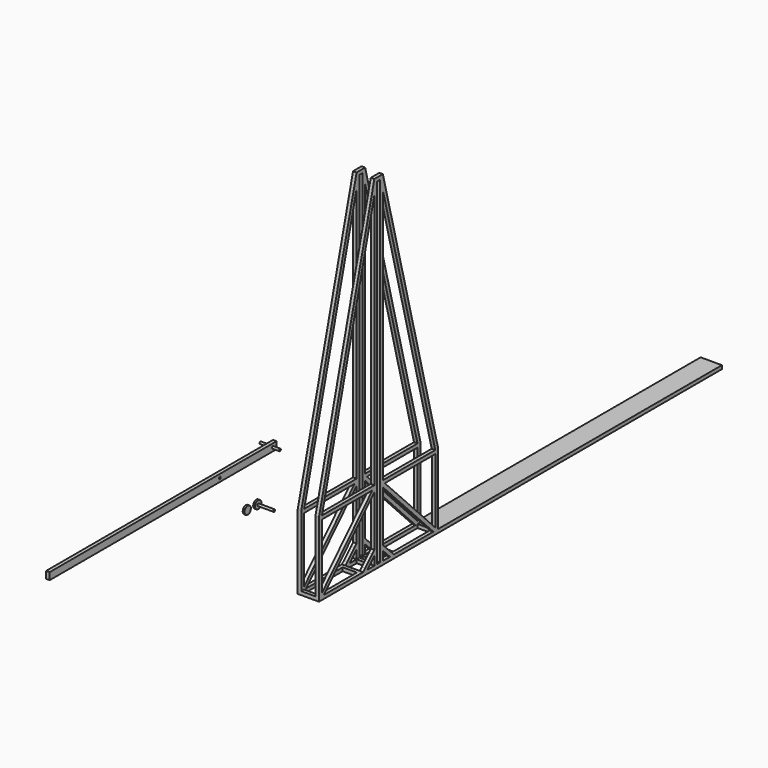
from build123d import *

# Parameters (mm, degrees)
F0_W      = 5.08
F0_H      = 5.08
F1_DEPTH  = 5.08
F4_W      = 5.08
F4_H      = 5.08
F5_DEPTH  = 20.32
F6_W      = 406.4
F6_H      = 10.16
F6_R      = 1.5875
F7_DEPTH  = 5.08
F8_R      = 5.715
F8_R_2    = 1.5875
F9_DEPTH  = 2.54
F10_DEPTH = 25.4
F11_R     = 5.715
F12_DEPTH = 2.54
F15_DEPTH = 15.24
F16_DEPTH = 12.7
F18_DEPTH = 508


# Not quite as in the source:
# - the program builds the solid bodies; features that only make, move or delete a surface that nothing else refers to are left out


with BuildPart() as f1:
    # F0 (on Right) → F1 (new body)
    with BuildSketch(Plane.YZ):
        Polygon((2.54, -101.6), (0, -101.6), (-2.54, -101.6), (-7.62, -101.6), (-20.32, -101.6), (-27.5042048969, -101.6), (-98.0548469748, -101.6), (-101.6, -101.6), (-101.6, -97.9590320281), (-101.6, -5.08), (-101.6, 0), (-106.68, 0), (-106.68, -106.68), (0, -106.68), (106.68, -106.68), (106.68, 0), (101.6, 0), (101.6, -5.08), (101.6, -97.9590320281), (101.6, -101.6), (98.0548469748, -101.6), (27.5042048969, -101.6), (20.32, -101.6), (7.62, -101.6), align=None)
        Polygon((101.4354498343, 0), (7.62, 0), (7.62, -5.08), (11.1651530252, -5.08), (101.6, -5.08), (101.6, 0), align=None)
        Polygon((-7.62, -5.08), (-7.62, 0), (-101.4354498343, 0), (-101.6, 0), (-101.6, -5.08), (-11.1651530252, -5.08), align=None)
        Polygon((2.54, 381), (2.54, 0), (7.62, 0), (7.62, 365.6397019183), (7.62, 381), align=None)
        Polygon((-7.62, 0), (-2.54, 0), (-2.54, 381), (-7.62, 381), (-7.62, 365.6397019183), align=None)
        Polygon((-2.54, 381), (2.54, 381), (7.62, 381), (7.62, 386.08), (-7.62, 386.08), (-7.62, 381), align=None)
        Polygon((-2.54, -101.6), (-2.54, -5.08), (-7.62, -5.08), (-7.62, -8.7209679719), (-7.62, -81.7157951031), (-7.62, -88.9), (-7.62, -101.6), align=None)
        Polygon((-7.62, -8.7209679719), (-7.62, -5.08), (-11.1651530252, -5.08), (-101.6, -97.9590320281), (-101.6, -101.6), (-98.0548469748, -101.6), align=None)
        with Locations((5.08, -2.54)):
            Rectangle(F0_W, F0_H)
        with Locations((-5.08, -2.54)):
            Rectangle(F0_W, F0_H)
        Polygon((7.62, -5.08), (2.54, -5.08), (2.54, -101.6), (7.62, -101.6), (7.62, -88.9), (7.62, -81.7157951031), (7.62, -8.7209679719), align=None)
        Polygon((11.1651530252, -5.08), (7.62, -5.08), (7.62, -8.7209679719), (98.0548469748, -101.6), (101.6, -101.6), (101.6, -97.9590320281), align=None)
        Polygon((11.2121024484, -85.3078975516), (7.62, -81.7157951031), (7.62, -88.9), (20.32, -101.6), (27.5042048969, -101.6), (23.9121024484, -98.0078975516), align=None)
        Polygon((-27.5042048969, -101.6), (-20.32, -101.6), (-7.62, -88.9), (-7.62, -81.7157951031), (-11.2121024484, -85.3078975516), (-23.9121024484, -98.0078975516), align=None)
        Polygon((7.62, 365.6397019183), (101.4354498343, 0), (101.6, 0), (106.68, 0), (7.62, 386.08), (7.62, 381), align=None)
        Polygon((-101.6, 0), (-101.4354498343, 0), (-7.62, 365.6397019183), (-7.62, 381), (-7.62, 386.08), (-106.68, 0), align=None)
    extrude(amount=F1_DEPTH)


with BuildPart() as f2_1:
    # F2: copy of F1
    add(f1.part)


with BuildPart() as f2_1_1:
    # F3: moved
    add(f2_1.part.moved(Location((-25.4, 0, 0))))


with BuildPart() as f1_1:
    add(f1.part)

    add(f2_1_1.part)  # F5 merges F2_1
    # F4 (on face) → F5 (join, through all)
    with BuildSketch(Plane(origin=(0, 0, 0), x_dir=(0, -1, 0), z_dir=(-1, 0, 0))):
        with Locations((-104.14, -104.14)):
            Rectangle(F4_W, F4_H)
        with Locations((-30.0442048969, -104.14)):
            Rectangle(F4_W, F4_H)
        with Locations((-5.08, -104.14)):
            Rectangle(F4_W, F4_H)
        with Locations((5.08, -104.14)):
            Rectangle(F4_W, F4_H)
        with Locations((30.0442048969, -104.14)):
            Rectangle(F4_W, F4_H)
        with Locations((104.14, -104.14)):
            Rectangle(F4_W, F4_H)
    extrude(amount=F5_DEPTH)

    # F17 (on face) → F18 (join)
    with BuildSketch(Plane(origin=(0, 106.68, 0), x_dir=(-1, 0, 0), z_dir=(0, 1, 0))):
        Polygon((0, -101.6), (-5.08, -101.6), (-5.08, -106.68), (25.4, -106.68), (25.4, -101.6), (20.32, -101.6), align=None)
    extrude(amount=F18_DEPTH)


with BuildPart() as f7:
    # F6 (on Right) → F7 (new body)
    with BuildSketch(Plane.YZ):
        with Locations((-385.7845490456, 121.5760712194)):
            Rectangle(F6_W, F6_H)
        with Locations((-284.1845490456, 121.5760712194)):
            Circle(F6_R, mode=Mode.SUBTRACT)
        with BuildLine():
            ThreePointArc((-190.8395490456, 121.5760712194), (-189.2520490456, 123.1635712194), (-187.6645490456, 121.5760712194))
            ThreePointArc((-187.6645490456, 121.5760712194), (-189.2520490456, 119.9885712194), (-190.8395490456, 121.5760712194))
        make_face(mode=Mode.SUBTRACT)
        with BuildLine():
            ThreePointArc((-190.8395490456, 121.5760712194), (-189.2520490456, 119.9885712194), (-187.6645490456, 121.5760712194))
            Line((-187.6645490456, 121.5760712194), (-190.8395490456, 121.5760712194))
        make_face()
        with BuildLine():
            Line((-190.8395490456, 121.5760712194), (-187.6645490456, 121.5760712194))
            ThreePointArc((-187.6645490456, 121.5760712194), (-189.2520490456, 123.1635712194), (-190.8395490456, 121.5760712194))
        make_face()
    extrude(amount=F7_DEPTH)

    # F6 (on Right) → F15 (join)
    with BuildSketch(Plane.YZ):
        with BuildLine():
            Line((-190.8395490456, 121.5760712194), (-187.6645490456, 121.5760712194))
            ThreePointArc((-187.6645490456, 121.5760712194), (-189.2520490456, 123.1635712194), (-190.8395490456, 121.5760712194))
        make_face()
        with BuildLine():
            ThreePointArc((-190.8395490456, 121.5760712194), (-189.2520490456, 119.9885712194), (-187.6645490456, 121.5760712194))
            Line((-187.6645490456, 121.5760712194), (-190.8395490456, 121.5760712194))
        make_face()
    extrude(amount=F15_DEPTH)

    # F6 (on Right) → F16 (join)
    with BuildSketch(Plane.YZ):
        with BuildLine():
            Line((-190.8395490456, 121.5760712194), (-187.6645490456, 121.5760712194))
            ThreePointArc((-187.6645490456, 121.5760712194), (-189.2520490456, 123.1635712194), (-190.8395490456, 121.5760712194))
        make_face()
        with BuildLine():
            ThreePointArc((-190.8395490456, 121.5760712194), (-189.2520490456, 119.9885712194), (-187.6645490456, 121.5760712194))
            Line((-187.6645490456, 121.5760712194), (-190.8395490456, 121.5760712194))
        make_face()
    extrude(amount=-F16_DEPTH)


with BuildPart() as f9:
    # F8 (on Right) → F9 (new body)
    with BuildSketch(Plane.YZ):
        with Locations((-212.4280929565, 57.8589513898)):
            Circle(F8_R)
        with Locations((-212.4280929565, 57.8589513898)):
            Circle(F8_R_2, mode=Mode.SUBTRACT)
        with Locations((-212.4280929565, 57.8589513898)):
            Circle(F8_R_2)
    extrude(amount=F9_DEPTH)

    # F8 (on Right) → F10 (join)
    with BuildSketch(Plane.YZ):
        with Locations((-212.4280929565, 57.8589513898)):
            Circle(F8_R_2)
    extrude(amount=F10_DEPTH)


with BuildPart() as f12:
    # F11 (on Right) → F12 (new body)
    with BuildSketch(Plane.YZ):
        with Locations((-231.2091737986, 58.4822148085)):
            Circle(F11_R)
    extrude(amount=F12_DEPTH)


solid = Compound([f1_1.part, f7.part, f9.part, f12.part])
